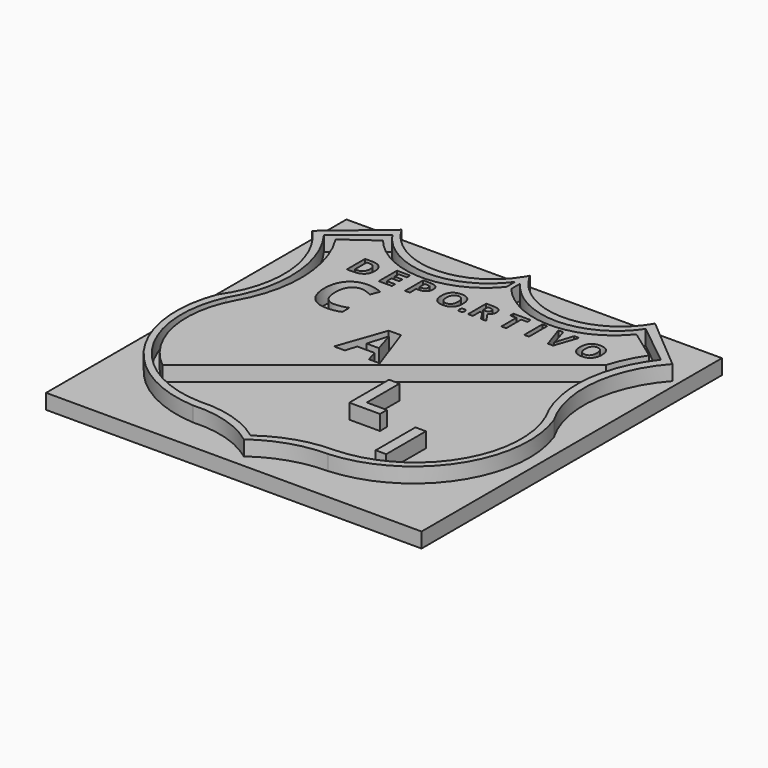
from build123d import *

# Parameters (mm, degrees)
F1_DEPTH       = 9
F2_W           = 225
F2_H           = 225
F3_DEPTH       = 9
F4_TEXT_SIZE   = 39.7433243635
F4_TEXT_SIZE_2 = 41.6666666667
F4_TEXT_SIZE_3 = 19.1258915092
F5_DEPTH       = 9
F6_TEXT_SIZE   = 41.6666666667
F7_DEPTH       = 9


# Not quite as in the source:
# - Text() gives the source's letters only with a copy of the font that has no kerning and outlines rounded to 1/6400 em; it was checked with that copy


with BuildPart() as f1:
    # F0 (on Top) → F1 (new body)
    with BuildSketch(Plane.XY):
        with BuildLine():
            ThreePointArc((-96.2868072869, 1.9591267182), (-86.306437991, 41.5427673925), (-100, 80))
            Line((-100, 80), (-75, 100))
            ThreePointArc((-75, 100), (-38.0426221222, 80.0043411209), (-0.5404601645, 98.9585491528))
            Line((-0.5404601645, 98.9585491528), (-0.5404601645, 105.5549174827))
            ThreePointArc((-0.5404601645, 105.5549174827), (-38.1830224324, 85.0078578199), (-75, 107))
            Line((-75, 107), (-107, 80))
            ThreePointArc((-107, 80), (-90.1139403523, 42.0066280762), (-101.2868072869, 1.9591267182))
            ThreePointArc((-101.2868072869, 1.9591267182), (-94.765947419, -61.0891738728), (-40, -93))
            ThreePointArc((-40, -93), (-18.9349229389, -95.4497431296), (0, -105))
            ThreePointArc((0, -105), (18.9610979577, -95.3033783314), (40, -92))
            ThreePointArc((40, -92), (93.8196888723, -60.8289823926), (101.0881339, 0.9396257823))
            ThreePointArc((101.0881339, 0.9396257823), (92.1142694694, 41.6867929321), (108.957277363, 79.8597540256))
            Line((108.957277363, 79.8597540256), (76.957277363, 106.8597540256))
            ThreePointArc((76.957277363, 106.8597540256), (40.0887272507, 84.8663968492), (2.4595398355, 105.5313914473))
            Line((2.4595398355, 105.5313914473), (2.4595398355, 98.939114988))
            ThreePointArc((2.4595398355, 98.939114988), (39.949836808, 79.8631617782), (76.957277363, 99.8597540256))
            Line((76.957277363, 99.8597540256), (101.957277363, 79.8597540256))
            ThreePointArc((101.957277363, 79.8597540256), (87.0491863443, 41.2901383107), (96.0881339, 0.9396257823))
            ThreePointArc((96.0881339, 0.9396257823), (91.2049473756, -57.8022600054), (40, -87))
            ThreePointArc((40, -87), (18.9610979577, -90.3033783314), (0, -100))
            ThreePointArc((0, -100), (-18.9349229389, -90.4497431296), (-40, -88))
            ThreePointArc((-40, -88), (-92.2123432126, -58.0802067004), (-96.2868072869, 1.9591267182))
        make_face()
        with BuildLine():
            Line((-0.5404601645, 105.5549174827), (-0.5404601645, 98.9585491528))
            Line((-0.5404601645, 98.9585491528), (-0.5404601645, 92.3379768727))
            ThreePointArc((-0.5404601645, 92.3379768727), (-37.9273089662, 75.0018995741), (-75, 93))
            Line((-75, 93), (-93, 80))
            ThreePointArc((-93, 80), (-81.2669047759, 41.2183297621), (-91.2868072869, 1.9591267182))
            ThreePointArc((-91.2868072869, 1.9591267182), (-96.9473729564, -36.5092641297), (-76.957277363, -69.8597540256))
            Line((-76.957277363, -69.8597540256), (85.236366937, 59.589112139))
            ThreePointArc((85.236366937, 59.589112139), (89.3376201982, 70.0885130265), (94.957277363, 79.8597540256))
            Line((94.957277363, 79.8597540256), (76.957277363, 92.8597540256))
            ThreePointArc((76.957277363, 92.8597540256), (39.8546886439, 74.8613970781), (2.4595398355, 92.2437383494))
            Line((2.4595398355, 92.2437383494), (2.4595398355, 98.939114988))
            Line((2.4595398355, 98.939114988), (2.4595398355, 105.5313914473))
            ThreePointArc((2.4595398355, 105.5313914473), (1.6859990758, 106.8490071848), (0.9595398355, 108.1931550602))
            ThreePointArc((0.9595398355, 108.1931550602), (0.2327004429, 106.8608680445), (-0.5404601645, 105.5549174827))
        make_face()
    extrude(amount=F1_DEPTH)

    # F2 (on face) → F3 (join)
    with BuildSketch(Plane(origin=(0, 0, 0), x_dir=(1, 0, 0), z_dir=(0, 0, -1))):
        Rectangle(F2_W, F2_H)
    extrude(amount=F3_DEPTH)

    # F4 (on face) → F5 (cut)
    with BuildSketch(Plane.XY.offset(9)):
        with Locations((-25.860455213, -5.1353209433)):
            Text('A', F4_TEXT_SIZE, font='Open Sans', font_style=FontStyle.BOLD, text_align=(TextAlign.LEFT, TextAlign.BOTTOM))
        with Locations((-68.6469135464, 23.4798725984)):
            Text('C', F4_TEXT_SIZE_2, font='Open Sans', font_style=FontStyle.BOLD, text_align=(TextAlign.LEFT, TextAlign.BOTTOM))
        with Locations((14.139544787, -45.1353209433)):
            Text('L', F4_TEXT_SIZE_2, font='Open Sans', font_style=FontStyle.BOLD, text_align=(TextAlign.LEFT, TextAlign.BOTTOM))
        with Locations((53.9572531203, -75.1353209433)):
            Text('I', F4_TEXT_SIZE_2, font='Open Sans', font_style=FontStyle.BOLD, text_align=(TextAlign.LEFT, TextAlign.BOTTOM))
        with Locations((0.9595398355, 59.589112139)):
            Text('R T I V O', F4_TEXT_SIZE_3, font='Open Sans', font_style=FontStyle.BOLD, text_align=(TextAlign.LEFT, TextAlign.BOTTOM))
        with Locations((-71.6531026474, 59.589112139)):
            Text('D E P O.', F4_TEXT_SIZE_3, font='Open Sans', font_style=FontStyle.BOLD, text_align=(TextAlign.LEFT, TextAlign.BOTTOM))
    extrude(amount=-F5_DEPTH, mode=Mode.SUBTRACT)

    # F6 (on face) → F7 (join)
    with BuildSketch(Plane.XY):
        with Locations((11.5624385978, -45.1353209433)):
            Text('L', F6_TEXT_SIZE, font='Open Sans', font_style=FontStyle.BOLD, text_align=(TextAlign.LEFT, TextAlign.BOTTOM))
        with Locations((51.3801469311, -75.1353209433)):
            Text('I', F6_TEXT_SIZE, font='Open Sans', font_style=FontStyle.BOLD, text_align=(TextAlign.LEFT, TextAlign.BOTTOM))
    extrude(amount=F7_DEPTH)


solid = f1.part
